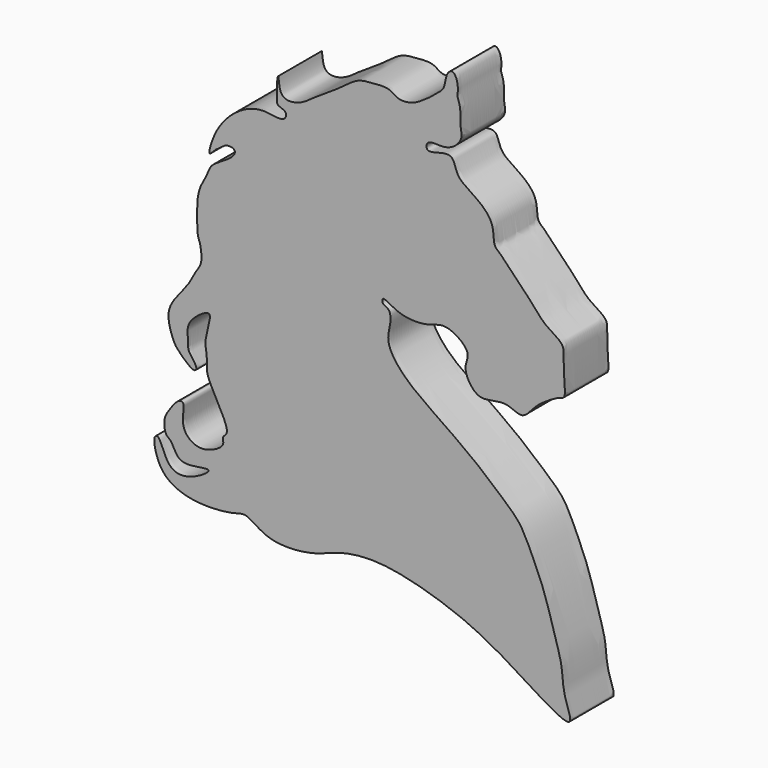
from build123d import *

# Parameters (mm, degrees)
F1_DEPTH = 5


with BuildPart() as f1:
    # F0 (on Front) → F1 (new body)
    with BuildSketch(Plane.XZ):
        with BuildLine():
            add(Edge.make_bspline(
                [(-11.3981273025, 5.9844749048), (-11.1560299541, 6.2011744716), (-12.0524642396, 8.077920231), (-11.9783511179, 10.2534779723), (-12.8551731683, 12.7603678187), (-13.581469782, 15.6152986354), (-14.8704525068, 18.4272659514), (-15.8505249491, 20.6074504017), (-17.5813777248, 22.1036913493), (-20.0285364305, 24.2681943136), (-23.6145134062, 26.7579046661), (-26.6227198306, 28.7960182303), (-28.3449487577, 31.229448503), (-27.7547142245, 32.7853200568), (-27.8398583271, 34.0077032953), (-28.6004008658, 34.0994542754), (-28.6115528349, 34.949962633), (-27.0393117177, 33.6571467644), (-24.2411899352, 33.709483894), (-22.7719462578, 34.6143873447), (-20.2142289631, 32.8717582895), (-21.3207774476, 31.5255363619), (-20.0786618354, 29.4785977177), (-18.7402205768, 29.5474422734), (-17.1006020771, 29.9847351718), (-15.7020485766, 28.9434773114), (-14.693734503, 30.337585281), (-13.7294088621, 31.0946522848), (-12.3642573738, 31.9358732166), (-11.6830940649, 31.9450652112), (-11.932268971, 33.8958216822), (-11.9220979664, 35.3898036967), (-11.9270303775, 36.1819258175), (-12.5823215854, 36.7497548657), (-13.753304362, 37.3422165288), (-15.0357167805, 38.9669365865), (-15.5699619466, 39.4307248485), (-17.6637798738, 41.7692022131), (-18.4001757807, 42.2017376227), (-18.3103696332, 43.7976486534), (-19.1714984864, 45.0047905349), (-20.5568746331, 45.9310582046), (-21.8360456265, 46.7532895101), (-21.9951359348, 48.4608678564), (-23.5425863505, 48.0472664884), (-24.581109195, 47.77261332), (-24.5168460165, 48.8899093769), (-22.8902841202, 48.5241650042), (-21.6899744091, 49.1599025045), (-21.1879293328, 50.0869709356), (-21.4717539993, 50.8385188066), (-21.3213444596, 52.4179605361), (-21.7415700708, 53.2014612611), (-21.5909742434, 53.6340008905), (-21.7006749871, 54.6791672306), (-22.198856199, 55.2149247815), (-22.7816119097, 54.6222437914), (-22.7765463372, 53.4700284072), (-23.6104005789, 52.7744423215), (-24.5902104436, 51.9888412503), (-25.8903708863, 51.181357716), (-27.2560854036, 51.1677228841), (-27.8630441836, 51.8847089083), (-29.7187746482, 51.7166864178), (-30.9794431525, 51.5922049407), (-32.6375739498, 50.1844551457), (-34.6270567821, 49.0470813833), (-35.903481869, 47.9385718035), (-37.5944155916, 47.6366038514), (-38.0788292724, 48.5327803032), (-38.1075000147, 49.737175629), (-38.2863502716, 48.9966208857), (-38.1592528902, 47.8426834018), (-38.370887596, 47.0348817201), (-37.2537441074, 46.9326815273), (-37.5639545281, 45.8225021687), (-39.5023028816, 46.4654317885), (-41.512928982, 45.7791042937), (-43.1262943213, 44.371441361), (-44.1127845643, 42.776175352), (-44.6809454459, 40.741086669), (-43.9238805229, 41.686741026), (-43.4449541179, 41.936003241), (-42.9302876753, 42.4385283944), (-42.0013453709, 42.3064931982), (-42.2071435209, 41.5506029405), (-43.5740784736, 40.7790026264), (-44.4036788591, 40.2218751351), (-44.6504079291, 39.3270638791), (-45.1991603883, 38.5134417594), (-45.5702379691, 37.3756732158), (-45.618589371, 35.8157719812), (-45.563333496, 34.1111593427), (-45.2888347258, 33.6962084846), (-45.0493085017, 32.0671488442), (-45.6790043824, 31.3447997041), (-46.1806543561, 30.1809615314), (-47.3622870276, 28.7731409085), (-48.597191684, 27.0860037568), (-47.7243377573, 24.8383596152), (-47.4275039401, 24.4483639197), (-46.9518145696, 23.9270557362), (-45.869026156, 22.9860205778), (-45.4952576306, 23.5251901853), (-46.3510799733, 24.4689583382), (-46.4085784472, 24.8737305723), (-46.4393785426, 25.4753058141), (-46.4614671675, 25.9872486331), (-46.4936789079, 27.0999401163), (-44.3679927742, 28.6249495398), (-44.4030553565, 27.5368819228), (-44.9682112531, 25.7973508198), (-44.6181294226, 24.8550662102), (-44.8050623504, 23.3204043966), (-44.1067568883, 22.1595899023), (-43.707675148, 21.278453337), (-43.1434308467, 20.2898559966), (-42.64288063, 19.0281111188), (-43.3683486643, 18.6779467701), (-42.9738464642, 17.9921768458), (-44.1984987472, 17.2165248865), (-45.4603233215, 16.9733159662), (-46.5463762381, 17.5816225164), (-47.0619709492, 18.6759449713), (-46.6447406962, 20.3369042374), (-47.3578410257, 20.3255125875), (-48.0498168257, 19.3909584068), (-48.7364788625, 18.4052295759), (-48.4984999095, 17.0333445899), (-47.8713822463, 16.8544383973), (-47.3774240807, 15.1362521013), (-45.4532632549, 15.5261279827), (-44.1041188765, 15.6792643484), (-45.5718476331, 14.6070066696), (-47.3213771467, 14.1119021807), (-48.5145306257, 15.0124979427), (-49.0345631319, 16.9325443166), (-49.6211364484, 16.6435856833), (-49.3984243403, 15.2250594806), (-48.5536341475, 13.4630991993), (-45.8065146076, 12.3961418103), (-42.2715506515, 12.6865225395), (-41.0130761726, 13.2773815004), (-39.0709193387, 11.3947991581), (-34.7374948518, 11.7856860907), (-32.5842127953, 12.915230569), (-28.7848952064, 13.4402957095), (-23.2755850862, 12.0269165547), (-18.9519792568, 10.2078942492), (-15.2015743319, 7.7956264948), (-11.731257391, 5.6862925981), (-11.3981273025, 5.9844749048)],
                knots=[0, 0, 0, 0, 0.0078904989, 0.0167269768, 0.0258357064, 0.0356830577, 0.0457173709, 0.0543939699, 0.0628053237, 0.0730944823, 0.0850687743, 0.0961096533, 0.1053992582, 0.1125210585, 0.1182795362, 0.1227130039, 0.1262152711, 0.1332048882, 0.1427654237, 0.1501139868, 0.1588347973, 0.1653616143, 0.1733659546, 0.1796823955, 0.186983703, 0.1937145212, 0.2003851469, 0.2070557738, 0.2141295277, 0.218033034, 0.2255081793, 0.2327999197, 0.2375603046, 0.2425104555, 0.2491929977, 0.2571203749, 0.262419633, 0.272291518, 0.2775430327, 0.2842379935, 0.2911028282, 0.2984571206, 0.3054027953, 0.3118904423, 0.3184724249, 0.3237776391, 0.3280806525, 0.3348362061, 0.3414729016, 0.346906586, 0.3519104771, 0.3590582619, 0.364206735, 0.3679306247, 0.3737343181, 0.377957453, 0.3824028619, 0.3883915526, 0.3941206285, 0.4005470313, 0.4076171747, 0.4139039256, 0.4191133346, 0.4265887538, 0.4330567376, 0.4412825998, 0.4499883219, 0.4574806392, 0.4643112441, 0.4698274872, 0.4750129163, 0.4784626733, 0.4849625938, 0.4895694623, 0.4946305939, 0.4990852306, 0.5066069082, 0.5149297013, 0.5230995192, 0.5314102024, 0.5380532869, 0.5426106736, 0.5471320811, 0.5518566522, 0.5566374524, 0.5607247071, 0.5678838163, 0.5735811336, 0.5788486886, 0.5844492335, 0.5905696836, 0.5978938169, 0.6051065463, 0.6092421744, 0.6161909007, 0.621689518, 0.6279570289, 0.635709372, 0.6438128826, 0.6521774326, 0.6560891652, 0.660986074, 0.6674159123, 0.6706532024, 0.6768286126, 0.6806169332, 0.6848647558, 0.6889107495, 0.694860467, 0.7029705449, 0.707254679, 0.7150294705, 0.7207570652, 0.7276333074, 0.7341729093, 0.7397245592, 0.7459729542, 0.7521587158, 0.7563857161, 0.7605366985, 0.7668771363, 0.7733900599, 0.7793779017, 0.7856414001, 0.7924787882, 0.7959719781, 0.8020144373, 0.8083960389, 0.8145706708, 0.8188676355, 0.8256400455, 0.8333939765, 0.8384690787, 0.8447265696, 0.8524709927, 0.8592039716, 0.8666915, 0.8697323814, 0.87616305, 0.8840086294, 0.8936247184, 0.9042758361, 0.9104504679, 0.9191256989, 0.930699185, 0.9396335299, 0.95046776, 0.9640534653, 0.9763352458, 0.9891425387, 1, 1, 1, 1], degree=3))
        make_face()
    extrude(amount=F1_DEPTH)


solid = f1.part
